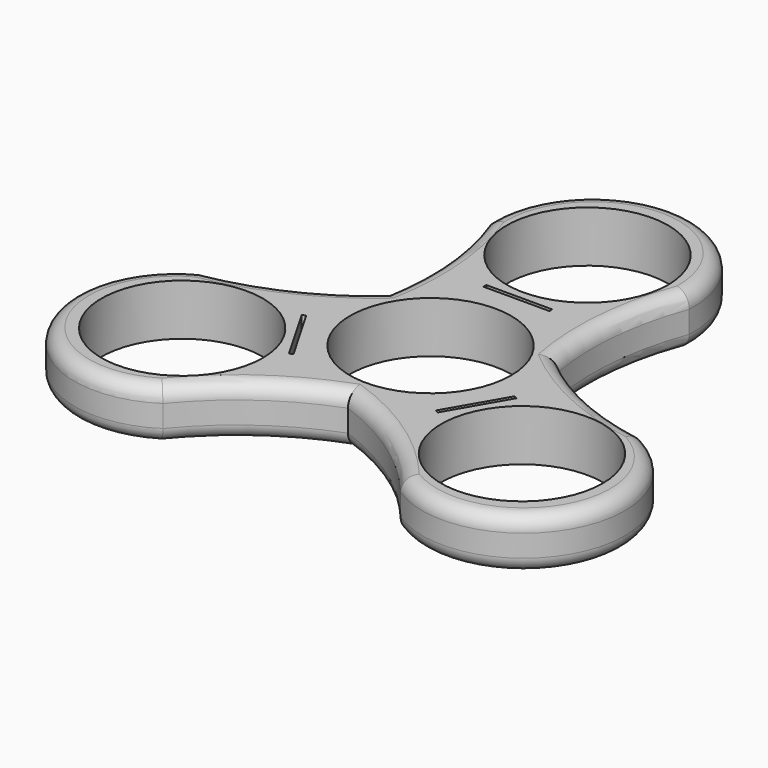
from build123d import *

# Parameters (mm, degrees)
F0_R         = 11
F0_W         = 9
F0_H         = 0.4958910868
F1_DEPTH     = 7
F2_T3_ANGLE  = 45.2058743493
F2_S4_R      = 38
F2_T5_DEPTH  = 19
F2_T8_ANGLE  = 227.522654694
F2_T11_ANGLE = 45.8937746322
F2_S12_R     = 38
F2_T13_DEPTH = 20
F2_T16_ANGLE = 45.2058743493
F2_S17_R     = 38
F2_T18_DEPTH = 20
F2_T21_ANGLE = 227.522654694
F2_T24_ANGLE = 45.8937746322
F2_S25_R     = 38
F2_T26_DEPTH = 21
F2_T29_ANGLE = 45.2058743493
F2_S30_R     = 38
F2_T31_DEPTH = 21
F2_T34_ANGLE = 227.522654694
F2_T37_ANGLE = 45.8937746322
F2_S38_R     = 38
F2_T39_DEPTH = 20
F2_T43_ANGLE = 45.2058743493
F2_S44_R     = 38
F2_T45_DEPTH = 19
F2_T48_ANGLE = 45.8937746322
F2_S49_R     = 38
F2_T50_DEPTH = 20
F2_T55_ANGLE = 45.8937746322
F2_S56_R     = 38
F2_T57_DEPTH = 20
F2_T60_ANGLE = 45.2058743493
F2_S61_R     = 38
F2_T62_DEPTH = 20
F2_T67_ANGLE = 45.2058743493
F2_S68_R     = 38
F2_T69_DEPTH = 21
F2_T72_ANGLE = 45.8937746322
F2_S73_R     = 38
F2_T74_DEPTH = 21
F3_T3_ANGLE  = 227.522654694
F3_T6_ANGLE  = 45.2058743493
F3_S7_R      = 38
F3_T8_DEPTH  = 19
F3_T11_ANGLE = 45.8937746322
F3_S12_R     = 38
F3_T13_DEPTH = 20
F3_T16_ANGLE = 227.522654694
F3_T19_ANGLE = 45.2058743493
F3_S20_R     = 38
F3_T21_DEPTH = 21
F3_T24_ANGLE = 45.8937746322
F3_S25_R     = 38
F3_T26_DEPTH = 21
F3_T29_ANGLE = 227.522654694
F3_T32_ANGLE = 45.2058743493
F3_S33_R     = 38
F3_T34_DEPTH = 20
F3_T37_ANGLE = 45.8937746322
F3_S38_R     = 38
F3_T39_DEPTH = 20
F3_T43_ANGLE = 45.8937746322
F3_S44_R     = 38
F3_T45_DEPTH = 20
F3_T48_ANGLE = 45.2058743493
F3_S49_R     = 38
F3_T50_DEPTH = 19
F3_T55_ANGLE = 45.8937746322
F3_S56_R     = 38
F3_T57_DEPTH = 21
F3_T60_ANGLE = 45.2058743493
F3_S61_R     = 38
F3_T62_DEPTH = 21
F3_T67_ANGLE = 45.8937746322
F3_S68_R     = 38
F3_T69_DEPTH = 20
F3_T72_ANGLE = 45.2058743493
F3_S73_R     = 38
F3_T74_DEPTH = 20


# Not quite as in the source:
# - a fillet or chamfer that OpenCascade refuses, or shapes differently, is made with other operations: its cross-section is extruded or revolved along the edge and cut away or added


with BuildPart() as f1:
    # F0 (on Top) → F1 (new body)
    with BuildSketch(Plane.XY):
        with BuildLine():
            ThreePointArc((12.0468410067, 6.6555924166), (11.6038749685, 16.833912258), (13.8810481876, 26.764113456))
            ThreePointArc((13.8810481876, 26.764113456), (0.0907252543, 41.2909770134), (-13.6995976791, 26.764113456))
            ThreePointArc((-13.6995976791, 26.764113456), (-11.4438268991, 17.0610116136), (-11.7873326133, 7.1050741388))
            ThreePointArc((-11.7873326133, 7.1050741388), (-20.3805331447, 1.6322943761), (-30.1189262565, -1.3607163664))
            ThreePointArc((-30.1189262565, -1.3607163664), (-35.8043976678, -20.5669181317), (-16.3286033231, -25.2462563397))
            ThreePointArc((-16.3286033231, -25.2462563397), (-9.053356022, -18.4411506179), (-0.2595083933, -13.7606665554))
            ThreePointArc((-0.2595083933, -13.7606665554), (8.7766581762, -18.466206634), (16.2378780689, -25.4033970896))
            ThreePointArc((16.2378780689, -25.4033970896), (35.7136724135, -20.7240588817), (30.0282010022, -1.5178571163))
            ThreePointArc((30.0282010022, -1.5178571163), (20.4971829212, 1.3801390044), (12.0468410067, 6.6555924166))
        make_face()
        with Locations((-23.1784021627, -13.382056728)):
            Circle(F0_R, mode=Mode.SUBTRACT)
        Polygon((-14.6960466328, -2.8242953981), (-10.1960466328, -10.6185240322), (-10.6255009115, -10.8664695756), (-15.1255009115, -3.0722409415), align=None, mode=Mode.SUBTRACT)
        with Locations((23.1784021627, -13.382056728)):
            Circle(F0_R, mode=Mode.SUBTRACT)
        Polygon((9.793934879, -11.3150020201), (14.293934879, -3.5207733861), (14.7233891576, -3.7687189295), (10.2233891576, -11.5629475635), align=None, mode=Mode.SUBTRACT)
        Circle(F0_R, mode=Mode.SUBTRACT)
        with Locations((0.4021117538, 14.3872429617)):
            Rectangle(F0_W, F0_H, mode=Mode.SUBTRACT)
        with Locations((0, 26.764113456)):
            Circle(F0_R, mode=Mode.SUBTRACT)
    extrude(amount=F1_DEPTH)

    # F2: fillet of radius 2 on 9 edges, made by hand


with BuildPart() as f2_tool1:
    # F2_s2 → F2_t3 (revolve)
    with BuildSketch(Plane(origin=(-16.5393520653, 30.8992120032, 0), x_dir=(0, 0, 1), z_dir=(-0.4719154962, 0.8816437855, 0))):
        with BuildLine():
            ThreePointArc((5, 0.8807372995), (6.4142135624, 1.4665237371), (7, 2.8807372995))
            Line((7, 2.8807372995), (7, 0.8807372995))
            Line((7, 0.8807372995), (5, 0.8807372995))
        make_face()
    revolve(axis=Axis((-49.2653193466, 13.382056728, 7), (0, 0, -1)), revolution_arc=F2_T3_ANGLE)

    # F2_s4 → F2_t5 (intersect, symmetric)
    with BuildSketch(Plane.XY.offset(5.3)):
        with Locations((-36.3125860089, 36.1311304656)):
            Circle(F2_S4_R)
    extrude(amount=F2_T5_DEPTH, both=True, mode=Mode.INTERSECT)


with BuildPart() as f2_tool6:
    # F2_s7 → F2_t8 (revolve)
    with BuildSketch(Plane(origin=(10.1493203818, 23.0537204739, 0), x_dir=(0, 0, 1), z_dir=(-0.4029276386, -0.9152318384, 0))):
        with BuildLine():
            ThreePointArc((5, -2.8187794742), (6.4142135624, -2.2329930365), (7, -0.8187794742))
            Line((7, -0.8187794742), (7, -2.8187794742))
            Line((7, -2.8187794742), (5, -2.8187794742))
        make_face()
    revolve(axis=Axis((0.0907252543, 27.4819820491, 7), (0, 0, 1)), revolution_arc=F2_T8_ANGLE)


with BuildPart() as f2_tool9:
    # F2_s10 → F2_t11 (revolve)
    with BuildSketch(Plane(origin=(0.7055478119, -2.2061129258, 0), x_dir=(0, 0, 1), z_dir=(0.3046158068, -0.9524753069, 0))):
        with BuildLine():
            ThreePointArc((5, -13.1732132997), (6.4142135624, -12.5874268621), (7, -11.1732132997))
            Line((7, -11.1732132997), (7, -13.1732132997))
            Line((7, -13.1732132997), (5, -13.1732132997))
        make_face()
    revolve(axis=Axis((49.4467698551, 13.382056728, 7), (0, 0, -1)), revolution_arc=F2_T11_ANGLE)

    # F2_s12 → F2_t13 (intersect, symmetric)
    with BuildSketch(Plane.XY.offset(5.3)):
        with Locations((36.2218607546, 35.9739897157)):
            Circle(F2_S12_R)
    extrude(amount=F2_T13_DEPTH, both=True, mode=Mode.INTERSECT)


with BuildPart() as f2_tool14:
    # F2_s15 → F2_t16 (revolve)
    with BuildSketch(Plane(origin=(35.0291785844, -1.1261069509, 0), x_dir=(0, 0, 1), z_dir=(0.9994836634, -0.0321310846, 0))):
        with BuildLine():
            ThreePointArc((5, 0.8807372995), (6.4142135624, 1.4665237371), (7, 2.8807372995))
            Line((7, 2.8807372995), (7, 0.8807372995))
            Line((7, 0.8807372995), (5, 0.8807372995))
        make_face()
    revolve(axis=Axis((36.2218607546, 35.9739897157, 7), (0, 0, -1)), revolution_arc=F2_T16_ANGLE)

    # F2_s17 → F2_t18 (intersect, symmetric)
    with BuildSketch(Plane.XY.offset(6)):
        with Locations((49.4467698551, 13.382056728)):
            Circle(F2_S17_R)
    extrude(amount=F2_T18_DEPTH, both=True, mode=Mode.INTERSECT)


with BuildPart() as f2_tool19:
    # F2_s20 → F2_t21 (revolve)
    with BuildSketch(Plane(origin=(14.8904473912, -20.3164295188, 0), x_dir=(0, 0, 1), z_dir=(-0.5911502031, 0.8065614901, 0))):
        with BuildLine():
            ThreePointArc((5, -2.8187794742), (6.4142135624, -2.2329930365), (7, -0.8187794742))
            Line((7, -0.8187794742), (7, -2.8187794742))
            Line((7, -2.8187794742), (5, -2.8187794742))
        make_face()
    revolve(axis=Axis((23.7547319738, -13.8195613995, 7), (0, 0, 1)), revolution_arc=F2_T21_ANGLE)


with BuildPart() as f2_tool22:
    # F2_s23 → F2_t24 (revolve)
    with BuildSketch(Plane(origin=(-2.2633237433, 0.4920341342, 0), x_dir=(0, 0, 1), z_dir=(-0.9771757156, 0.2124326264, 0))):
        with BuildLine():
            ThreePointArc((5, -13.1732132997), (6.4142135624, -12.5874268621), (7, -11.1732132997))
            Line((7, -11.1732132997), (7, -13.1732132997))
            Line((7, -13.1732132997), (5, -13.1732132997))
        make_face()
    revolve(axis=Axis((-13.1341838462, -49.5131871936, 7), (0, 0, -1)), revolution_arc=F2_T24_ANGLE)

    # F2_s25 → F2_t26 (intersect, symmetric)
    with BuildSketch(Plane.XY.offset(6)):
        with Locations((13.0434585919, -49.3560464437)):
            Circle(F2_S25_R)
    extrude(amount=F2_T26_DEPTH, both=True, mode=Mode.INTERSECT)


with BuildPart() as f2_tool27:
    # F2_s28 → F2_t29 (revolve)
    with BuildSketch(Plane(origin=(-18.4898265191, -29.7731050523, 0), x_dir=(0, 0, 1), z_dir=(-0.5275681672, -0.8495127009, 0))):
        with BuildLine():
            ThreePointArc((5, 0.8807372995), (6.4142135624, 1.4665237371), (7, 2.8807372995))
            Line((7, 2.8807372995), (7, 0.8807372995))
            Line((7, 0.8807372995), (5, 0.8807372995))
        make_face()
    revolve(axis=Axis((13.0434585919, -49.3560464437, 7), (0, 0, -1)), revolution_arc=F2_T29_ANGLE)

    # F2_s30 → F2_t31 (intersect, symmetric)
    with BuildSketch(Plane.XY.offset(5.3)):
        with Locations((-13.1341838462, -49.5131871936)):
            Circle(F2_S30_R)
    extrude(amount=F2_T31_DEPTH, both=True, mode=Mode.INTERSECT)


with BuildPart() as f2_tool32:
    # F2_s33 → F2_t34 (revolve)
    with BuildSketch(Plane(origin=(-25.0397677731, -2.7372909551, 0), x_dir=(0, 0, 1), z_dir=(0.9940778417, 0.1086703483, 0))):
        with BuildLine():
            ThreePointArc((5, -2.8187794742), (6.4142135624, -2.2329930365), (7, -0.8187794742))
            Line((7, -0.8187794742), (7, -2.8187794742))
            Line((7, -2.8187794742), (5, -2.8187794742))
        make_face()
    revolve(axis=Axis((-23.845457228, -13.6624206496, 7), (0, 0, 1)), revolution_arc=F2_T34_ANGLE)


with BuildPart() as f2_tool35:
    # F2_s36 → F2_t37 (revolve)
    with BuildSketch(Plane(origin=(1.5577759314, 1.7140787916, 0), x_dir=(0, 0, 1), z_dir=(0.6725599089, 0.7400426805, 0))):
        with BuildLine():
            ThreePointArc((5, -13.1732132997), (6.4142135624, -12.5874268621), (7, -11.1732132997))
            Line((7, -11.1732132997), (7, -13.1732132997))
            Line((7, -13.1732132997), (5, -13.1732132997))
        make_face()
    revolve(axis=Axis((-36.3125860089, 36.1311304656, 7), (0, 0, -1)), revolution_arc=F2_T37_ANGLE)

    # F2_s38 → F2_t39 (intersect, symmetric)
    with BuildSketch(Plane.XY.offset(6)):
        with Locations((-49.2653193466, 13.382056728)):
            Circle(F2_S38_R)
    extrude(amount=F2_T39_DEPTH, both=True, mode=Mode.INTERSECT)


with BuildPart() as f2_tool41:
    # F2_s42 → F2_t43 (revolve)
    with BuildSketch(Plane(origin=(-16.5393520653, 30.8992120032, 0), x_dir=(0, 0, 1), z_dir=(-0.4719154962, 0.8816437855, 0))):
        with BuildLine():
            ThreePointArc((5, 0.8807372995), (6.4142135624, 1.4665237371), (7, 2.8807372995))
            Line((7, 2.8807372995), (7, 0.8807372995))
            Line((7, 0.8807372995), (5, 0.8807372995))
        make_face()
    revolve(axis=Axis((-49.2653193466, 13.382056728, 7), (0, 0, -1)), revolution_arc=F2_T43_ANGLE)

    # F2_s44 → F2_t45 (cut, symmetric)
    with BuildSketch(Plane.XY.offset(5.3)):
        with Locations((-36.3125860089, 36.1311304656)):
            Circle(F2_S44_R)
    extrude(amount=F2_T45_DEPTH, both=True, mode=Mode.SUBTRACT)


with BuildPart() as f2_tool46:
    # F2_s47 → F2_t48 (revolve)
    with BuildSketch(Plane(origin=(1.5577759314, 1.7140787916, 0), x_dir=(0, 0, 1), z_dir=(0.6725599089, 0.7400426805, 0))):
        with BuildLine():
            ThreePointArc((5, -13.1732132997), (6.4142135624, -12.5874268621), (7, -11.1732132997))
            Line((7, -11.1732132997), (7, -13.1732132997))
            Line((7, -13.1732132997), (5, -13.1732132997))
        make_face()
    revolve(axis=Axis((-36.3125860089, 36.1311304656, 7), (0, 0, -1)), revolution_arc=F2_T48_ANGLE)

    # F2_s49 → F2_t50 (cut, symmetric)
    with BuildSketch(Plane.XY.offset(6)):
        with Locations((-49.2653193466, 13.382056728)):
            Circle(F2_S49_R)
    extrude(amount=F2_T50_DEPTH, both=True, mode=Mode.SUBTRACT)


with BuildPart() as f2_tool41_1:
    add(f2_tool41.part)

    # F2_t51: intersect F2_tool46
    add(f2_tool46.part, mode=Mode.INTERSECT)


with BuildPart() as f2_tool53:
    # F2_s54 → F2_t55 (revolve)
    with BuildSketch(Plane(origin=(0.7055478119, -2.2061129258, 0), x_dir=(0, 0, 1), z_dir=(0.3046158068, -0.9524753069, 0))):
        with BuildLine():
            ThreePointArc((5, -13.1732132997), (6.4142135624, -12.5874268621), (7, -11.1732132997))
            Line((7, -11.1732132997), (7, -13.1732132997))
            Line((7, -13.1732132997), (5, -13.1732132997))
        make_face()
    revolve(axis=Axis((49.4467698551, 13.382056728, 7), (0, 0, -1)), revolution_arc=F2_T55_ANGLE)

    # F2_s56 → F2_t57 (cut, symmetric)
    with BuildSketch(Plane.XY.offset(5.3)):
        with Locations((36.2218607546, 35.9739897157)):
            Circle(F2_S56_R)
    extrude(amount=F2_T57_DEPTH, both=True, mode=Mode.SUBTRACT)


with BuildPart() as f2_tool58:
    # F2_s59 → F2_t60 (revolve)
    with BuildSketch(Plane(origin=(35.0291785844, -1.1261069509, 0), x_dir=(0, 0, 1), z_dir=(0.9994836634, -0.0321310846, 0))):
        with BuildLine():
            ThreePointArc((5, 0.8807372995), (6.4142135624, 1.4665237371), (7, 2.8807372995))
            Line((7, 2.8807372995), (7, 0.8807372995))
            Line((7, 0.8807372995), (5, 0.8807372995))
        make_face()
    revolve(axis=Axis((36.2218607546, 35.9739897157, 7), (0, 0, -1)), revolution_arc=F2_T60_ANGLE)

    # F2_s61 → F2_t62 (cut, symmetric)
    with BuildSketch(Plane.XY.offset(6)):
        with Locations((49.4467698551, 13.382056728)):
            Circle(F2_S61_R)
    extrude(amount=F2_T62_DEPTH, both=True, mode=Mode.SUBTRACT)


with BuildPart() as f2_tool53_1:
    add(f2_tool53.part)

    # F2_t63: intersect F2_tool58
    add(f2_tool58.part, mode=Mode.INTERSECT)


with BuildPart() as f2_tool65:
    # F2_s66 → F2_t67 (revolve)
    with BuildSketch(Plane(origin=(-18.4898265191, -29.7731050523, 0), x_dir=(0, 0, 1), z_dir=(-0.5275681672, -0.8495127009, 0))):
        with BuildLine():
            ThreePointArc((5, 0.8807372995), (6.4142135624, 1.4665237371), (7, 2.8807372995))
            Line((7, 2.8807372995), (7, 0.8807372995))
            Line((7, 0.8807372995), (5, 0.8807372995))
        make_face()
    revolve(axis=Axis((13.0434585919, -49.3560464437, 7), (0, 0, -1)), revolution_arc=F2_T67_ANGLE)

    # F2_s68 → F2_t69 (cut, symmetric)
    with BuildSketch(Plane.XY.offset(5.3)):
        with Locations((-13.1341838462, -49.5131871936)):
            Circle(F2_S68_R)
    extrude(amount=F2_T69_DEPTH, both=True, mode=Mode.SUBTRACT)


with BuildPart() as f2_tool70:
    # F2_s71 → F2_t72 (revolve)
    with BuildSketch(Plane(origin=(-2.2633237433, 0.4920341342, 0), x_dir=(0, 0, 1), z_dir=(-0.9771757156, 0.2124326264, 0))):
        with BuildLine():
            ThreePointArc((5, -13.1732132997), (6.4142135624, -12.5874268621), (7, -11.1732132997))
            Line((7, -11.1732132997), (7, -13.1732132997))
            Line((7, -13.1732132997), (5, -13.1732132997))
        make_face()
    revolve(axis=Axis((-13.1341838462, -49.5131871936, 7), (0, 0, -1)), revolution_arc=F2_T72_ANGLE)

    # F2_s73 → F2_t74 (cut, symmetric)
    with BuildSketch(Plane.XY.offset(6)):
        with Locations((13.0434585919, -49.3560464437)):
            Circle(F2_S73_R)
    extrude(amount=F2_T74_DEPTH, both=True, mode=Mode.SUBTRACT)


with BuildPart() as f2_tool65_1:
    add(f2_tool65.part)

    # F2_t75: intersect F2_tool70
    add(f2_tool70.part, mode=Mode.INTERSECT)


with BuildPart() as f1_1:
    add(f1.part)

    # F2_t76: cut F2_tool1, F2_tool6, F2_tool9, F2_tool14, F2_tool19, F2_tool22, F2_tool27, F2_tool32, F2_tool35, F2_tool41, F2_tool53, F2_tool65
    add([f2_tool1.part, f2_tool6.part, f2_tool9.part, f2_tool14.part, f2_tool19.part, f2_tool22.part, f2_tool27.part, f2_tool32.part, f2_tool35.part, f2_tool41_1.part, f2_tool53_1.part, f2_tool65_1.part], mode=Mode.SUBTRACT)

    # F3: fillet of radius 2 on 9 edges, made by hand


with BuildPart() as f3_tool1:
    # F3_s2 → F3_t3 (revolve)
    with BuildSketch(Plane(origin=(10.1493203818, 23.0537204739, 0), x_dir=(0, 0, 1), z_dir=(-0.4029276386, -0.9152318384, 0))):
        with BuildLine():
            ThreePointArc((2, -2.8187794742), (0.5857864376, -2.2329930365), (0, -0.8187794742))
            Line((0, -0.8187794742), (0, -2.8187794742))
            Line((0, -2.8187794742), (2, -2.8187794742))
        make_face()
    revolve(axis=Axis((0.0907252543, 27.4819820491, 0), (0, 0, 1)), revolution_arc=F3_T3_ANGLE)


with BuildPart() as f3_tool4:
    # F3_s5 → F3_t6 (revolve)
    with BuildSketch(Plane(origin=(-16.5393520653, 30.8992120032, 0), x_dir=(0, 0, 1), z_dir=(-0.4719154962, 0.8816437855, 0))):
        with BuildLine():
            ThreePointArc((2, 0.8807372995), (0.5857864376, 1.4665237371), (0, 2.8807372995))
            Line((0, 2.8807372995), (0, 0.8807372995))
            Line((0, 0.8807372995), (2, 0.8807372995))
        make_face()
    revolve(axis=Axis((-49.2653193466, 13.382056728, 0), (0, 0, -1)), revolution_arc=F3_T6_ANGLE)

    # F3_s7 → F3_t8 (intersect, symmetric)
    with BuildSketch(Plane.XY.offset(1.7)):
        with Locations((-36.3125860089, 36.1311304656)):
            Circle(F3_S7_R)
    extrude(amount=F3_T8_DEPTH, both=True, mode=Mode.INTERSECT)


with BuildPart() as f3_tool9:
    # F3_s10 → F3_t11 (revolve)
    with BuildSketch(Plane(origin=(1.5577759314, 1.7140787916, 0), x_dir=(0, 0, 1), z_dir=(0.6725599089, 0.7400426805, 0))):
        with BuildLine():
            ThreePointArc((2, -13.1732132997), (0.5857864376, -12.5874268621), (0, -11.1732132997))
            Line((0, -11.1732132997), (0, -13.1732132997))
            Line((0, -13.1732132997), (2, -13.1732132997))
        make_face()
    revolve(axis=Axis((-36.3125860089, 36.1311304656, 0), (0, 0, -1)), revolution_arc=F3_T11_ANGLE)

    # F3_s12 → F3_t13 (intersect, symmetric)
    with BuildSketch(Plane.XY.offset(1)):
        with Locations((-49.2653193466, 13.382056728)):
            Circle(F3_S12_R)
    extrude(amount=F3_T13_DEPTH, both=True, mode=Mode.INTERSECT)


with BuildPart() as f3_tool14:
    # F3_s15 → F3_t16 (revolve)
    with BuildSketch(Plane(origin=(-25.0397677731, -2.7372909551, 0), x_dir=(0, 0, 1), z_dir=(0.9940778417, 0.1086703483, 0))):
        with BuildLine():
            ThreePointArc((2, -2.8187794742), (0.5857864376, -2.2329930365), (0, -0.8187794742))
            Line((0, -0.8187794742), (0, -2.8187794742))
            Line((0, -2.8187794742), (2, -2.8187794742))
        make_face()
    revolve(axis=Axis((-23.845457228, -13.6624206496, 0), (0, 0, 1)), revolution_arc=F3_T16_ANGLE)


with BuildPart() as f3_tool17:
    # F3_s18 → F3_t19 (revolve)
    with BuildSketch(Plane(origin=(-18.4898265191, -29.7731050523, 0), x_dir=(0, 0, 1), z_dir=(-0.5275681672, -0.8495127009, 0))):
        with BuildLine():
            ThreePointArc((2, 0.8807372995), (0.5857864376, 1.4665237371), (0, 2.8807372995))
            Line((0, 2.8807372995), (0, 0.8807372995))
            Line((0, 0.8807372995), (2, 0.8807372995))
        make_face()
    revolve(axis=Axis((13.0434585919, -49.3560464437, 0), (0, 0, -1)), revolution_arc=F3_T19_ANGLE)

    # F3_s20 → F3_t21 (intersect, symmetric)
    with BuildSketch(Plane.XY.offset(1.7)):
        with Locations((-13.1341838462, -49.5131871936)):
            Circle(F3_S20_R)
    extrude(amount=F3_T21_DEPTH, both=True, mode=Mode.INTERSECT)


with BuildPart() as f3_tool22:
    # F3_s23 → F3_t24 (revolve)
    with BuildSketch(Plane(origin=(-2.2633237433, 0.4920341342, 0), x_dir=(0, 0, 1), z_dir=(-0.9771757156, 0.2124326264, 0))):
        with BuildLine():
            ThreePointArc((2, -13.1732132997), (0.5857864376, -12.5874268621), (0, -11.1732132997))
            Line((0, -11.1732132997), (0, -13.1732132997))
            Line((0, -13.1732132997), (2, -13.1732132997))
        make_face()
    revolve(axis=Axis((-13.1341838462, -49.5131871936, 0), (0, 0, -1)), revolution_arc=F3_T24_ANGLE)

    # F3_s25 → F3_t26 (intersect, symmetric)
    with BuildSketch(Plane.XY.offset(1.7)):
        with Locations((13.0434585919, -49.3560464437)):
            Circle(F3_S25_R)
    extrude(amount=F3_T26_DEPTH, both=True, mode=Mode.INTERSECT)


with BuildPart() as f3_tool27:
    # F3_s28 → F3_t29 (revolve)
    with BuildSketch(Plane(origin=(14.8904473912, -20.3164295188, 0), x_dir=(0, 0, 1), z_dir=(-0.5911502031, 0.8065614901, 0))):
        with BuildLine():
            ThreePointArc((2, -2.8187794742), (0.5857864376, -2.2329930365), (0, -0.8187794742))
            Line((0, -0.8187794742), (0, -2.8187794742))
            Line((0, -2.8187794742), (2, -2.8187794742))
        make_face()
    revolve(axis=Axis((23.7547319738, -13.8195613995, 0), (0, 0, 1)), revolution_arc=F3_T29_ANGLE)


with BuildPart() as f3_tool30:
    # F3_s31 → F3_t32 (revolve)
    with BuildSketch(Plane(origin=(35.0291785844, -1.1261069509, 0), x_dir=(0, 0, 1), z_dir=(0.9994836634, -0.0321310846, 0))):
        with BuildLine():
            ThreePointArc((2, 0.8807372995), (0.5857864376, 1.4665237371), (0, 2.8807372995))
            Line((0, 2.8807372995), (0, 0.8807372995))
            Line((0, 0.8807372995), (2, 0.8807372995))
        make_face()
    revolve(axis=Axis((36.2218607546, 35.9739897157, 0), (0, 0, -1)), revolution_arc=F3_T32_ANGLE)

    # F3_s33 → F3_t34 (intersect, symmetric)
    with BuildSketch(Plane.XY.offset(1)):
        with Locations((49.4467698551, 13.382056728)):
            Circle(F3_S33_R)
    extrude(amount=F3_T34_DEPTH, both=True, mode=Mode.INTERSECT)


with BuildPart() as f3_tool35:
    # F3_s36 → F3_t37 (revolve)
    with BuildSketch(Plane(origin=(0.7055478119, -2.2061129258, 0), x_dir=(0, 0, 1), z_dir=(0.3046158068, -0.9524753069, 0))):
        with BuildLine():
            ThreePointArc((2, -13.1732132997), (0.5857864376, -12.5874268621), (0, -11.1732132997))
            Line((0, -11.1732132997), (0, -13.1732132997))
            Line((0, -13.1732132997), (2, -13.1732132997))
        make_face()
    revolve(axis=Axis((49.4467698551, 13.382056728, 0), (0, 0, -1)), revolution_arc=F3_T37_ANGLE)

    # F3_s38 → F3_t39 (intersect, symmetric)
    with BuildSketch(Plane.XY.offset(1.7)):
        with Locations((36.2218607546, 35.9739897157)):
            Circle(F3_S38_R)
    extrude(amount=F3_T39_DEPTH, both=True, mode=Mode.INTERSECT)


with BuildPart() as f3_tool41:
    # F3_s42 → F3_t43 (revolve)
    with BuildSketch(Plane(origin=(1.5577759314, 1.7140787916, 0), x_dir=(0, 0, 1), z_dir=(0.6725599089, 0.7400426805, 0))):
        with BuildLine():
            ThreePointArc((2, -13.1732132997), (0.5857864376, -12.5874268621), (0, -11.1732132997))
            Line((0, -11.1732132997), (0, -13.1732132997))
            Line((0, -13.1732132997), (2, -13.1732132997))
        make_face()
    revolve(axis=Axis((-36.3125860089, 36.1311304656, 0), (0, 0, -1)), revolution_arc=F3_T43_ANGLE)

    # F3_s44 → F3_t45 (cut, symmetric)
    with BuildSketch(Plane.XY.offset(1)):
        with Locations((-49.2653193466, 13.382056728)):
            Circle(F3_S44_R)
    extrude(amount=F3_T45_DEPTH, both=True, mode=Mode.SUBTRACT)


with BuildPart() as f3_tool46:
    # F3_s47 → F3_t48 (revolve)
    with BuildSketch(Plane(origin=(-16.5393520653, 30.8992120032, 0), x_dir=(0, 0, 1), z_dir=(-0.4719154962, 0.8816437855, 0))):
        with BuildLine():
            ThreePointArc((2, 0.8807372995), (0.5857864376, 1.4665237371), (0, 2.8807372995))
            Line((0, 2.8807372995), (0, 0.8807372995))
            Line((0, 0.8807372995), (2, 0.8807372995))
        make_face()
    revolve(axis=Axis((-49.2653193466, 13.382056728, 0), (0, 0, -1)), revolution_arc=F3_T48_ANGLE)

    # F3_s49 → F3_t50 (cut, symmetric)
    with BuildSketch(Plane.XY.offset(1.7)):
        with Locations((-36.3125860089, 36.1311304656)):
            Circle(F3_S49_R)
    extrude(amount=F3_T50_DEPTH, both=True, mode=Mode.SUBTRACT)


with BuildPart() as f3_tool41_1:
    add(f3_tool41.part)

    # F3_t51: intersect F3_tool46
    add(f3_tool46.part, mode=Mode.INTERSECT)


with BuildPart() as f3_tool53:
    # F3_s54 → F3_t55 (revolve)
    with BuildSketch(Plane(origin=(-2.2633237433, 0.4920341342, 0), x_dir=(0, 0, 1), z_dir=(-0.9771757156, 0.2124326264, 0))):
        with BuildLine():
            ThreePointArc((2, -13.1732132997), (0.5857864376, -12.5874268621), (0, -11.1732132997))
            Line((0, -11.1732132997), (0, -13.1732132997))
            Line((0, -13.1732132997), (2, -13.1732132997))
        make_face()
    revolve(axis=Axis((-13.1341838462, -49.5131871936, 0), (0, 0, -1)), revolution_arc=F3_T55_ANGLE)

    # F3_s56 → F3_t57 (cut, symmetric)
    with BuildSketch(Plane.XY.offset(1.7)):
        with Locations((13.0434585919, -49.3560464437)):
            Circle(F3_S56_R)
    extrude(amount=F3_T57_DEPTH, both=True, mode=Mode.SUBTRACT)


with BuildPart() as f3_tool58:
    # F3_s59 → F3_t60 (revolve)
    with BuildSketch(Plane(origin=(-18.4898265191, -29.7731050523, 0), x_dir=(0, 0, 1), z_dir=(-0.5275681672, -0.8495127009, 0))):
        with BuildLine():
            ThreePointArc((2, 0.8807372995), (0.5857864376, 1.4665237371), (0, 2.8807372995))
            Line((0, 2.8807372995), (0, 0.8807372995))
            Line((0, 0.8807372995), (2, 0.8807372995))
        make_face()
    revolve(axis=Axis((13.0434585919, -49.3560464437, 0), (0, 0, -1)), revolution_arc=F3_T60_ANGLE)

    # F3_s61 → F3_t62 (cut, symmetric)
    with BuildSketch(Plane.XY.offset(1.7)):
        with Locations((-13.1341838462, -49.5131871936)):
            Circle(F3_S61_R)
    extrude(amount=F3_T62_DEPTH, both=True, mode=Mode.SUBTRACT)


with BuildPart() as f3_tool53_1:
    add(f3_tool53.part)

    # F3_t63: intersect F3_tool58
    add(f3_tool58.part, mode=Mode.INTERSECT)


with BuildPart() as f3_tool65:
    # F3_s66 → F3_t67 (revolve)
    with BuildSketch(Plane(origin=(0.7055478119, -2.2061129258, 0), x_dir=(0, 0, 1), z_dir=(0.3046158068, -0.9524753069, 0))):
        with BuildLine():
            ThreePointArc((2, -13.1732132997), (0.5857864376, -12.5874268621), (0, -11.1732132997))
            Line((0, -11.1732132997), (0, -13.1732132997))
            Line((0, -13.1732132997), (2, -13.1732132997))
        make_face()
    revolve(axis=Axis((49.4467698551, 13.382056728, 0), (0, 0, -1)), revolution_arc=F3_T67_ANGLE)

    # F3_s68 → F3_t69 (cut, symmetric)
    with BuildSketch(Plane.XY.offset(1.7)):
        with Locations((36.2218607546, 35.9739897157)):
            Circle(F3_S68_R)
    extrude(amount=F3_T69_DEPTH, both=True, mode=Mode.SUBTRACT)


with BuildPart() as f3_tool70:
    # F3_s71 → F3_t72 (revolve)
    with BuildSketch(Plane(origin=(35.0291785844, -1.1261069509, 0), x_dir=(0, 0, 1), z_dir=(0.9994836634, -0.0321310846, 0))):
        with BuildLine():
            ThreePointArc((2, 0.8807372995), (0.5857864376, 1.4665237371), (0, 2.8807372995))
            Line((0, 2.8807372995), (0, 0.8807372995))
            Line((0, 0.8807372995), (2, 0.8807372995))
        make_face()
    revolve(axis=Axis((36.2218607546, 35.9739897157, 0), (0, 0, -1)), revolution_arc=F3_T72_ANGLE)

    # F3_s73 → F3_t74 (cut, symmetric)
    with BuildSketch(Plane.XY.offset(1)):
        with Locations((49.4467698551, 13.382056728)):
            Circle(F3_S73_R)
    extrude(amount=F3_T74_DEPTH, both=True, mode=Mode.SUBTRACT)


with BuildPart() as f3_tool65_1:
    add(f3_tool65.part)

    # F3_t75: intersect F3_tool70
    add(f3_tool70.part, mode=Mode.INTERSECT)


with BuildPart() as f1_2:
    add(f1_1.part)

    # F3_t76: cut F3_tool1, F3_tool4, F3_tool9, F3_tool14, F3_tool17, F3_tool22, F3_tool27, F3_tool30, F3_tool35, F3_tool41, F3_tool53, F3_tool65
    add([f3_tool1.part, f3_tool4.part, f3_tool9.part, f3_tool14.part, f3_tool17.part, f3_tool22.part, f3_tool27.part, f3_tool30.part, f3_tool35.part, f3_tool41_1.part, f3_tool53_1.part, f3_tool65_1.part], mode=Mode.SUBTRACT)


solid = f1_2.part
